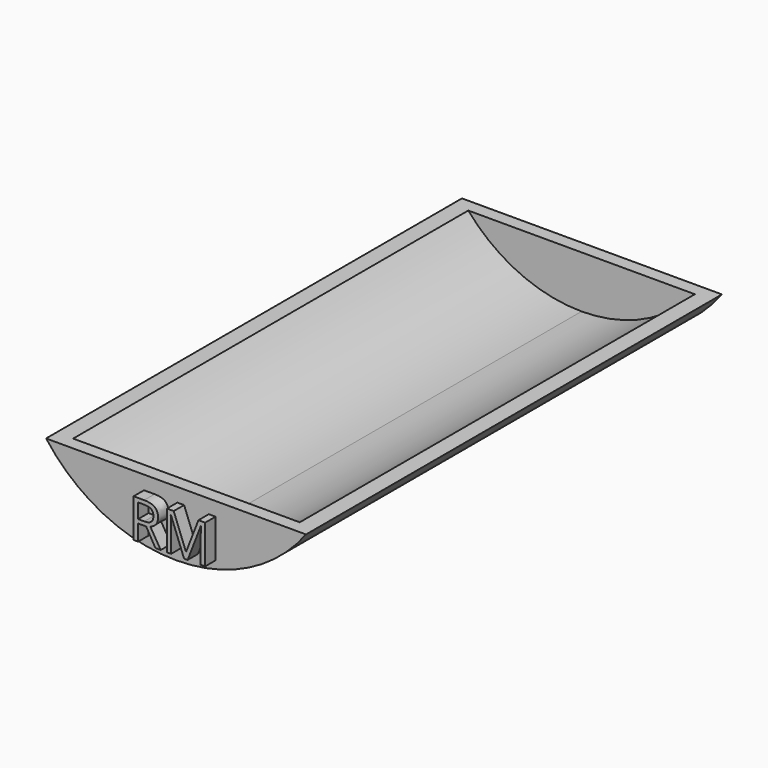
from build123d import *

# Parameters (mm, degrees)
F1_DEPTH     = 101.6
F2_T         = -2.54
F3_TEXT_SIZE = 10.5447058255
F4_DEPTH     = 2.54


# Not quite as in the source:
# - Text() gives the source's letters only with a copy of the font that has no kerning and outlines rounded to 1/6400 em; it was checked with that copy


with BuildPart() as f1:
    # F0 (on Front) → F1 (new body)
    with BuildSketch(Plane.XZ):
        with BuildLine():
            Line((0.7207474291, 39.2749793828), (-24.6792525709, 39.2749793828))
            Line((-24.6792525709, 39.2749793828), (-24.6792525709, 26.5749793828))
            ThreePointArc((-24.6792525709, 26.5749793828), (-10.4802209137, 29.9269160685), (0.7207474291, 39.2749793828))
        make_face()
        with BuildLine():
            Line((-24.6792525709, 39.2749793828), (-50.0792525709, 39.2749793828))
            ThreePointArc((-50.0792525709, 39.2749793828), (-38.878284228, 29.9269160685), (-24.6792525709, 26.5749793828))
            Line((-24.6792525709, 26.5749793828), (-24.6792525709, 39.2749793828))
        make_face()
    extrude(amount=F1_DEPTH)

    # F2
    f2_openings = [f1.faces().sort_by_distance(p)[0] for p in [
        (-24.679253, -50.8, 39.274979),
    ]]
    offset(amount=F2_T, openings=f2_openings)

    # F3 (on face) → F4 (join)
    with BuildSketch(Plane.XZ.offset(101.6)):
        with Locations((-31.9747980684, 29.0547255427)):
            Text('RM', F3_TEXT_SIZE, font='Open Sans', text_align=(TextAlign.LEFT, TextAlign.BOTTOM))
    extrude(amount=F4_DEPTH)


solid = f1.part
